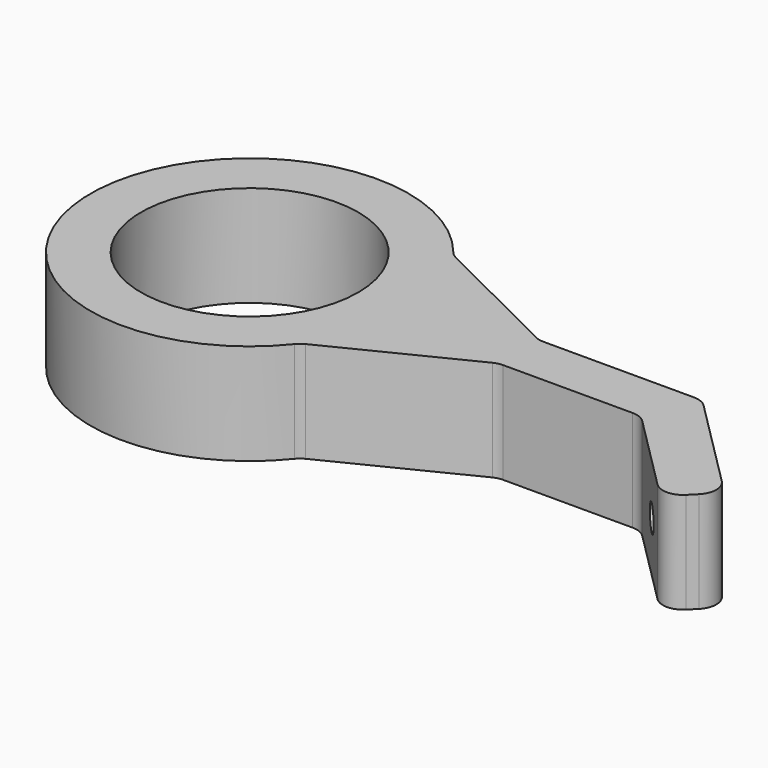
from build123d import *

# Parameters (mm, degrees)
F0_R        = 10.75
F1_DEPTH    = 10
F2_T1_DEPTH = 10
F3_R        = 1.31
F4_DEPTH    = 25
F5_R        = 2


# Not quite as in the source:
# - a fillet or chamfer that OpenCascade refuses, or shapes differently, is made with other operations: its cross-section is extruded or revolved along the edge and cut away or added


with BuildPart() as f1:
    # F0 (on Top) → F1 (new body)
    with BuildSketch(Plane.XY):
        with BuildLine():
            Line((40.75, 2.5), (15.5503215401, 2.5))
            ThreePointArc((15.5503215401, 2.5), (-15.75, 0), (15.5503215401, -2.5))
            Line((15.5503215401, -2.5), (40.75, -2.5))
            Line((40.75, -2.5), (50.295941546, -12.045941546))
            Line((50.295941546, -12.045941546), (53.831475452, -8.5104076401))
            Line((53.831475452, -8.5104076401), (42.8210678119, 2.5))
            Line((42.8210678119, 2.5), (40.75, 2.5))
        make_face()
        Circle(F0_R, mode=Mode.SUBTRACT)
    extrude(amount=F1_DEPTH)

    # F2: chamfer of 15 on 2 edges, made by hand

    # F2_s2 → F2_t1 (join)
    with BuildSketch(Plane.XY):
        with BuildLine():
            Line((27.1514391605, -2.2325951169), (12.0303066019, -9.7606848759))
            Line((12.0303066019, -9.7606848759), (11.7909271055, -9.579860495))
            ThreePointArc((11.7909271055, -9.579860495), (14.1178891417, -6.2759625701), (15.2541249393, -2.4523809524))
            Line((15.2541249393, -2.4523809524), (15.5503215401, -2.2))
            ThreePointArc((15.5503215401, -2.2), (21.3508803503, -2.2), (27.1514391605, -1.9325951169))
            Line((27.1514391605, -1.9325951169), (27.1514391605, -2.2325951169))
        make_face()
        with BuildLine():
            Line((12.0303066019, 9.7606848759), (27.1514391605, 2.2325951169))
            Line((27.1514391605, 2.2325951169), (27.1514391605, 1.9325951169))
            ThreePointArc((27.1514391605, 1.9325951169), (21.3508803503, 2.2), (15.5503215401, 2.2))
            Line((15.5503215401, 2.2), (15.2541249393, 2.4523809524))
            ThreePointArc((15.2541249393, 2.4523809524), (14.1178891417, 6.2759625701), (11.7909271055, 9.579860495))
            Line((11.7909271055, 9.579860495), (12.0303066019, 9.7606848759))
        make_face()
    extrude(amount=F2_T1_DEPTH)

    # F3 (on face) → F4 (cut)
    with BuildSketch(Plane(origin=(19.125, 19.125, 0), x_dir=(0.7071067812, -0.7071067812, 0), z_dir=(-0.7071067812, -0.7071067812, 0))):
        with Locations((38.0823682863, 5)):
            Circle(F3_R)
    extrude(amount=-F4_DEPTH, mode=Mode.SUBTRACT)

    # F5
    f5_edges = [f1.edges().sort_by_distance(p)[0] for p in [
        (50.295942, -12.045942, 5),
        (53.831475, -8.510408, 5),
        (40.75, -2.5, 5),
        (26.614322, -2.5, 5),
        (12.567424, -9.49328, 5),
        (42.821068, 2.5, 5),
        (26.614322, 2.5, 5),
        (12.567424, 9.49328, 5),
    ]]
    fillet(f5_edges, radius=F5_R)


solid = f1.part
